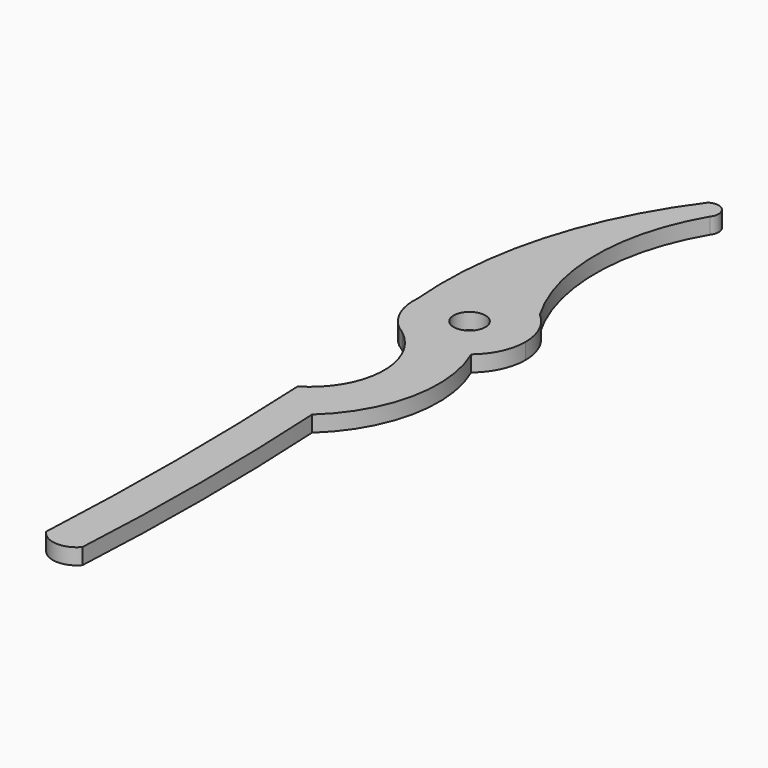
from build123d import *

# Parameters (mm, degrees)
F0_R     = 3.97
F1_DEPTH = 4


# Not quite as in the source:
# - a feature names something its author has since deleted; it is built from what else it names


with BuildPart() as f1:
    # F0 (on Top) → F1 (new body)
    with BuildSketch(Plane.XY):
        with BuildLine():
            ThreePointArc((-22.9417117699, 12), (-21.9452900598, 5.3928142737), (-18, 0))
            Line((-18, 0), (0, 0))
            ThreePointArc((0, 0), (3.6885775404, 4.8077255117), (5, 10.7238052948))
            ThreePointArc((5, 10.7238052948), (3.6885775404, 16.6398850779), (0, 21.4476105895))
            ThreePointArc((0, 21.4476105895), (-14.3309910211, 23.6690953546), (-22.9417117699, 12))
        make_face()
        with Locations((-9, 10.7238052948)):
            Circle(F0_R, mode=Mode.SUBTRACT)
        with BuildLine():
            ThreePointArc((-16.0404020707, -1.3771342837), (-9.1181835678, -17.0975519696), (-18, -31.8))
            ThreePointArc((-18, -31.8), (-16.9964304208, -71.1), (-18, -110.4))
            ThreePointArc((-18, -110.4), (-13.3652762377, -113.1756773925), (-8.3776302295, -111.1))
            ThreePointArc((-8.3776302295, -111.1), (-7.3699541271, -75.2), (-8.3776302295, -39.3))
            ThreePointArc((-8.3776302295, -39.3), (2.1233033288, -20.9955621955), (0, 0))
            ThreePointArc((0, 0), (-7.8024480304, -3.2248817144), (-16.0404020707, -1.3771342837))
        make_face()
        with BuildLine():
            ThreePointArc((-18, 0), (-16.9980479925, -0.6570443939), (-16.0404020707, -1.3771342837))
            ThreePointArc((-16.0404020707, -1.3771342837), (-7.8024480304, -3.2248817144), (0, 0))
            Line((0, 0), (-18, 0))
        make_face()
        with BuildLine():
            ThreePointArc((-4.0337323592, 79), (-19.6376277503, 47.2355565684), (-22.9417117699, 12))
            ThreePointArc((-22.9417117699, 12), (-14.3309910211, 23.6690953546), (0, 21.4476105895))
            ThreePointArc((0, 21.4476105895), (-7.2455477856, 48.0476105895), (0, 74.6476105895))
            ThreePointArc((0, 74.6476105895), (-0.1415918591, 78.5617827585), (-4.0337323592, 79))
        make_face()
    extrude(amount=F1_DEPTH)


solid = f1.part
